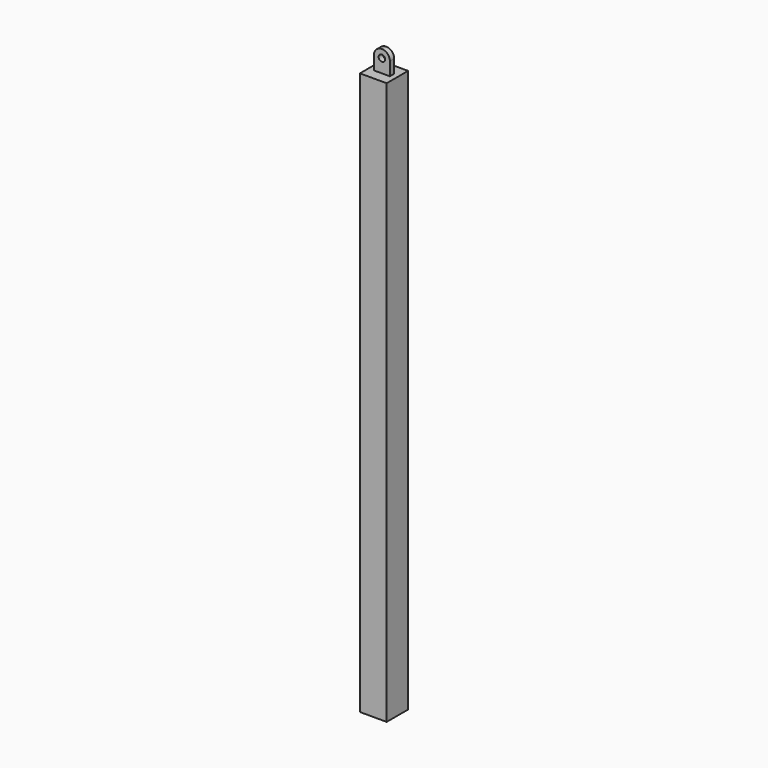
from build123d import *

# Parameters (mm, degrees)
F0_W     = 31.75
F0_H     = 666.75
F1_DEPTH = 31.75
F2_W     = 19.05
F2_H     = 6.35
F3_DEPTH = 25.4
F4_R     = 9.52499
F5_R     = 3.81
F6_DEPTH = 6.35


# Not quite as in the source:
# - a fillet or chamfer is up to 0.001 mm smaller than in the source, because OpenCascade refuses the exact size


with BuildPart() as f1:
    # F0 (on Front) → F1 (new body)
    with BuildSketch(Plane.XZ):
        with Locations((-15.875, 127.5886728781)):
            Rectangle(F0_W, F0_H)
    extrude(amount=-F1_DEPTH)

    # F2 (on face) → F3 (join)
    with BuildSketch(Plane.XY.offset(460.9636728781)):
        with Locations((-15.875, 15.875)):
            Rectangle(F2_W, F2_H)
    extrude(amount=F3_DEPTH)

    # F4 (radius 9.525 in the source; OpenCascade refuses exactly that, so slightly less here)
    f4_edges = [f1.edges().sort_by_distance(p)[0] for p in [
        (-6.35, 15.875, 486.363673),
        (-25.4, 15.875, 486.363673),
    ]]
    fillet(f4_edges, radius=F4_R)

    # F5 (on face) → F6 (cut)
    with BuildSketch(Plane.XZ.offset(-12.7)):
        with Locations((-15.875, 476.8386728781)):
            Circle(F5_R)
    extrude(amount=-F6_DEPTH, mode=Mode.SUBTRACT)


solid = f1.part
